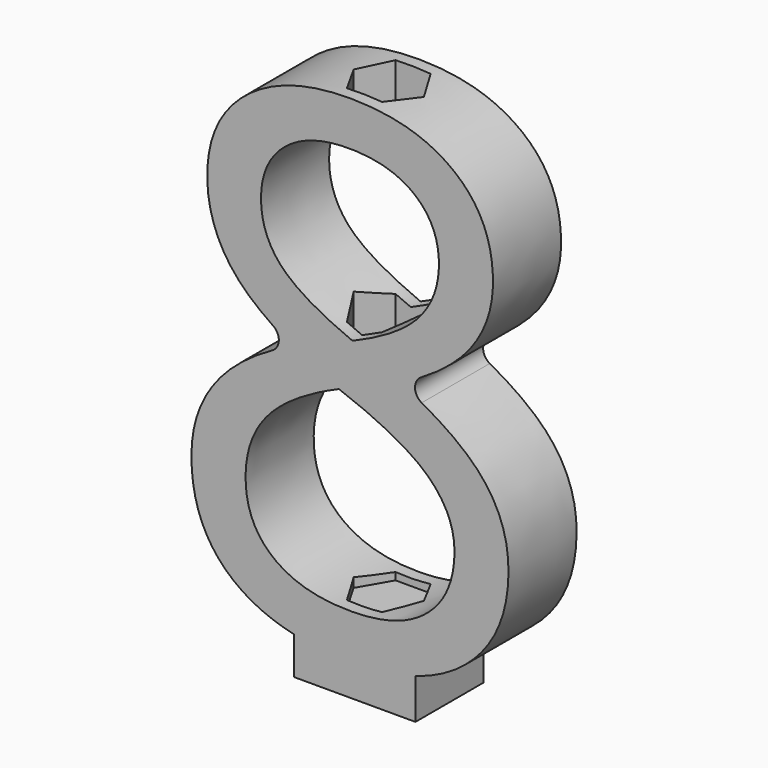
from build123d import *

# Parameters (mm, degrees)
F0_TEXT_SIZE  = 70.5555555556
F1_DEPTH      = 8.89
F4_DEPTH      = 47.8536
F5_R          = 1.3452512448
F7_W          = 6.35
F7_H          = 8.89
F8_DEPTH      = 2.7178
F8_DEPTH_BACK = 3.3274


# Not quite as in the source:
# - Text() gives the source's letters only with a copy of the font that has no kerning and outlines rounded to 1/6400 em; it was checked with that copy


with BuildPart() as f1:
    # F0 (on Front) → F1 (new body)
    with BuildSketch(Plane.XZ):
        with Locations((0, 0)):
            Text('8', F0_TEXT_SIZE, font='Open Sans', text_align=(TextAlign.LEFT, TextAlign.BOTTOM))
    extrude(amount=F1_DEPTH)

    # F3 (on plane+point) → F4 (cut)
    with BuildSketch(Plane.XY.offset(51.0866319444)):
        Polygon((20.6319882, -7.62), (20.6319882, -1.27), (18.7989010953, -1.27), (16.9658139906, -4.445), (18.7989010953, -7.62), align=None)
        Polygon((22.4650753047, -1.27), (20.6319882, -1.27), (20.6319882, -7.62), (22.4650753047, -7.62), (24.2981624094, -4.445), align=None)
    extrude(amount=-F4_DEPTH, mode=Mode.SUBTRACT)

    # F5
    f5_edges = [f1.edges().sort_by_distance(p)[0] for p in [
        (14.122135, -4.445, 26.326042),
        (25.388976, -4.445, 26.667795),
    ]]
    fillet(f5_edges, radius=F5_R)

    # F7 (on plane+point) → F8 (join, two sides)
    with BuildSketch(Plane.XY.offset(-0.69453125)) as f8_sk:
        with Locations((17.4498, -4.445)):
            Rectangle(F7_W, F7_H)
        with Locations((23.7998, -4.445)):
            Rectangle(F7_W, F7_H)
    extrude(amount=F8_DEPTH)
    extrude(f8_sk.sketch, amount=-F8_DEPTH_BACK)


solid = f1.part
